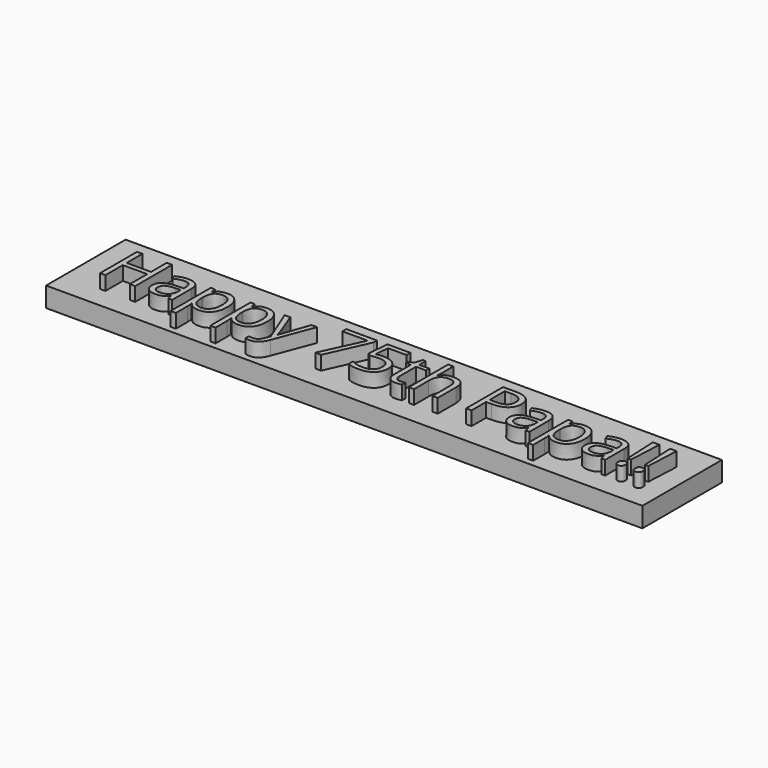
from build123d import *

# Parameters (mm, degrees)
F1_TEXT_SIZE = 8.2743581182
F2_DEPTH     = 1.778
F0_W         = 76.2
F0_H         = 12.7
F3_DEPTH     = 2.54


# Not quite as in the source:
# - Text() gives the source's letters only with a copy of the font that has no kerning and outlines rounded to 1/6400 em; it was checked with that copy


with BuildPart() as f2:
    # F1 (on face) → F2 (new body)
    with BuildSketch(Plane.XY):
        with Locations((0, 0)):
            Text('Happy 75th Papa!!', F1_TEXT_SIZE, font='Open Sans', text_align=(TextAlign.LEFT, TextAlign.BOTTOM))
    extrude(amount=F2_DEPTH)


with BuildPart() as f3:
    # F0 (on Top) → F3 (new body)
    with BuildSketch(Plane.XY):
        with Locations((34.2399531458, 3.5681039259)):
            Rectangle(F0_W, F0_H)
    extrude(amount=-F3_DEPTH)


solid = Compound([f2.part, f3.part])
